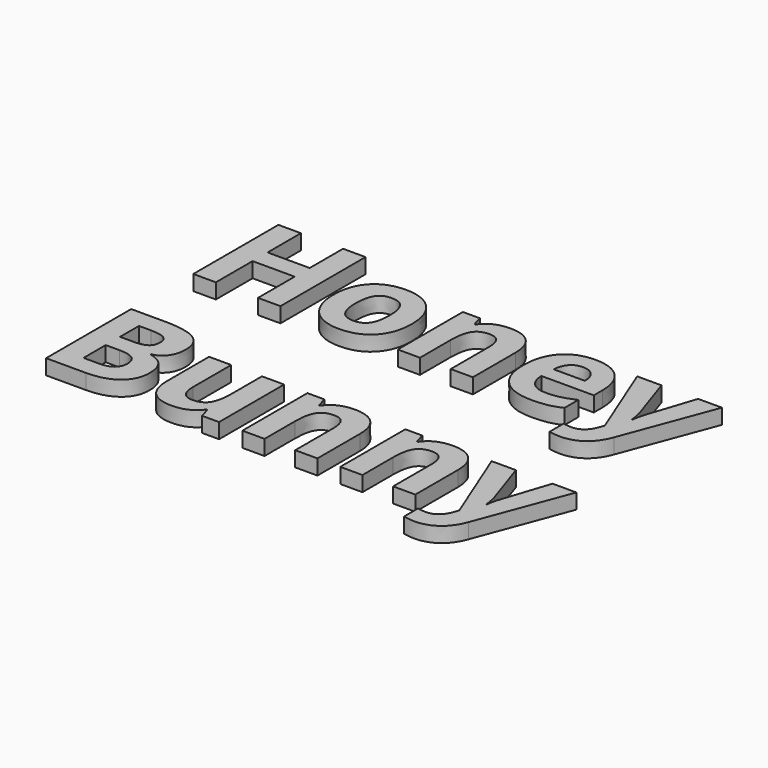
from build123d import *

# Parameters (mm, degrees)
F0_TEXT_SIZE = 11.8055555556
F2_DEPTH     = 1.2
F1_TEXT_SIZE = 11.8055555556
F3_DEPTH     = 1.2


# Not quite as in the source:
# - Text() gives the source's letters only with a copy of the font that has no kerning and outlines rounded to 1/6400 em; it was checked with that copy


with BuildPart() as f2:
    # F0 (on Top) → F2 (new body)
    with BuildSketch(Plane.XY):
        with Locations((-18.8962673611, 3)):
            Text('Honey', F0_TEXT_SIZE, font='Open Sans', font_style=FontStyle.BOLD, text_align=(TextAlign.LEFT, TextAlign.BOTTOM))
    extrude(amount=F2_DEPTH)


with BuildPart() as f3:
    # F1 (on Top) → F3 (new body)
    with BuildSketch(Plane.XY):
        with Locations((-18.9617513021, -11.5)):
            Text('Bunny', F1_TEXT_SIZE, font='Open Sans', font_style=FontStyle.BOLD, text_align=(TextAlign.LEFT, TextAlign.BOTTOM))
    extrude(amount=F3_DEPTH)


solid = Compound([f2.part, f3.part])
